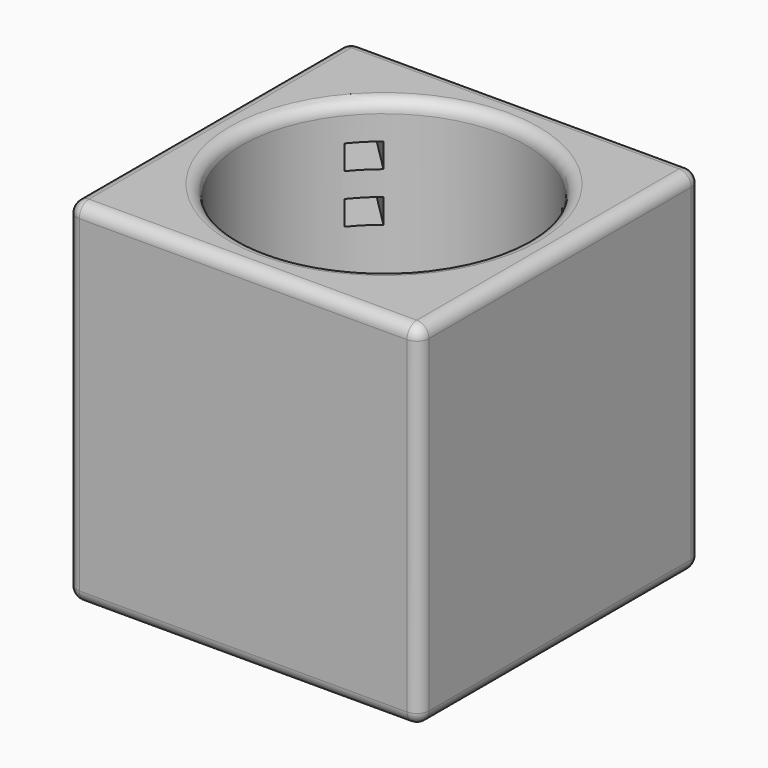
from build123d import *

# Parameters (mm, degrees)
F0_W     = 288
F0_H     = 288
F0_R     = 116.5
F1_DEPTH = 288
F2_R     = 10
F4_W     = 25
F4_H     = 20
F5_DEPTH = 166.5
F7_W     = 25
F7_H     = 20
F8_DEPTH = 166.5


with BuildPart() as f1:
    # F0 (on Top) → F1 (new body)
    with BuildSketch(Plane.XY):
        Rectangle(F0_W, F0_H)
        Circle(F0_R, mode=Mode.SUBTRACT)
    extrude(amount=F1_DEPTH)

    # F2
    f2_edges = [f1.edges().sort_by_distance(p)[0] for p in [
        (144, 0, 288),
        (0, 144, 288),
        (-144, 0, 288),
        (0, -144, 288),
        (-116.5, 0, 288),
        (144, 0, 0),
        (0, 144, 0),
        (-144, 0, 0),
        (0, -144, 0),
        (-116.5, 0, 0),
        (-144, 144, 144),
        (-144, -144, 144),
        (144, -144, 144),
        (144, 144, 144),
    ]]
    fillet(f2_edges, radius=F2_R)

    # F4 (on face) → F5 (cut, symmetric)
    with BuildSketch(Plane(origin=(0, 0, 0), x_dir=(-0.7071067812, 0.7071067812, 0), z_dir=(0.7071067812, 0.7071067812, 0))):
        with Locations((0, 248)):
            Rectangle(F4_W, F4_H)
        with Locations((0, 208)):
            Rectangle(F4_W, F4_H)
    extrude(amount=F5_DEPTH, both=True, mode=Mode.SUBTRACT)

    # F7 (on face) → F8 (cut, symmetric)
    with BuildSketch(Plane(origin=(0, 0, 0), x_dir=(0.7071067812, 0.7071067812, 0), z_dir=(0.7071067812, -0.7071067812, 0))):
        with Locations((0, 248)):
            Rectangle(F7_W, F7_H)
        with Locations((0, 208)):
            Rectangle(F7_W, F7_H)
    extrude(amount=F8_DEPTH, both=True, mode=Mode.SUBTRACT)


solid = f1.part
